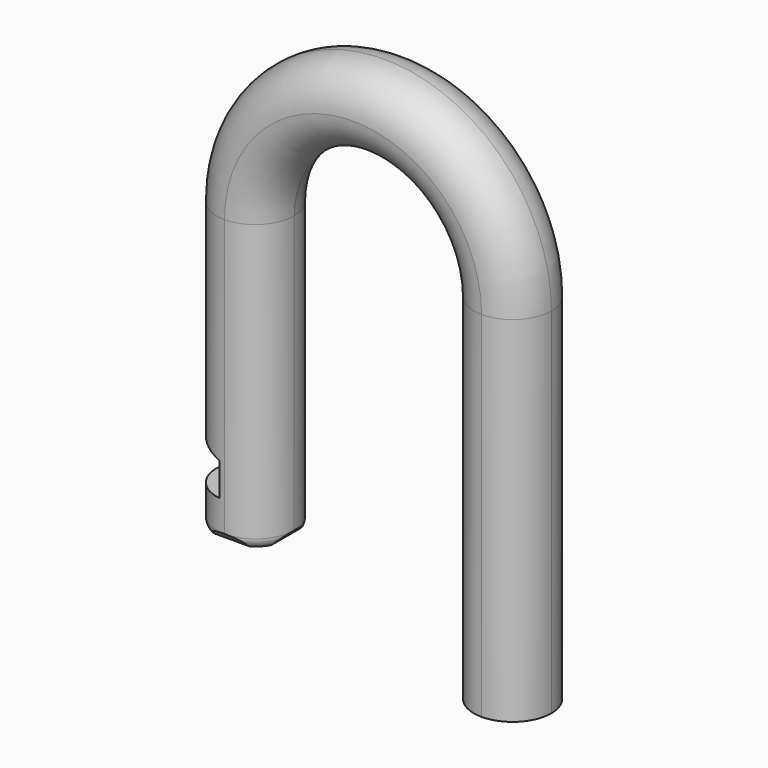
from build123d import *

# Parameters (mm, degrees)
F0_W         = 7
F0_H         = 1
F1_DEPTH     = 7
F2_SIZE      = 1
F3_T1_DEPTH  = 40.75
F3_T3_DEPTH  = 33.75
F3_T5_DEPTH  = 27.1711544693
F3_T8_ANGLE  = 180
F3_T10_ANGLE = 180
F3_T12_ANGLE = 180
F3_T14_ANGLE = 180
F4_R         = 0.99999


# Not quite as in the source:
# - a fillet or chamfer that OpenCascade refuses, or shapes differently, is made with other operations: its cross-section is extruded or revolved along the edge and cut away or added
# - a fillet or chamfer is up to 0.001 mm smaller than in the source, because OpenCascade refuses the exact size


with BuildPart() as f1:
    # F0 (on Front) → F1 (new body)
    with BuildSketch(Plane.XZ):
        with BuildLine():
            ThreePointArc((-8.115, 0), (0, 8.115), (8.115, 0))
            Line((8.115, 0), (8.115, -32))
            Line((8.115, -32), (15.115, -32))
            Line((15.115, -32), (15.115, 0))
            ThreePointArc((15.115, 0), (0, 15.115), (-15.115, 0))
            Line((-15.115, 0), (-15.115, -18.4211544693))
            Line((-15.115, -18.4211544693), (-12.115, -19.3215445876))
            Line((-12.115, -19.3215445876), (-12.115, -22.3215445876))
            Line((-12.115, -22.3215445876), (-15.115, -22.3215445876))
            Line((-15.115, -22.3215445876), (-15.115, -25))
            Line((-15.115, -25), (-8.115, -25))
            Line((-8.115, -25), (-8.115, 0))
        make_face()
        with Locations((-11.615, -25.5)):
            Rectangle(F0_W, F0_H)
    extrude(amount=-F1_DEPTH)

    # F2
    f2_edges = [f1.edges().sort_by_distance(p)[0] for p in [
        (-8.115, 3.5, -26),
        (-11.615, 0, -26),
        (-11.615, 7, -26),
        (-15.115, 3.5, -26),
    ]]
    chamfer(f2_edges, length=F2_SIZE)

    # F3: fillet of radius 3.5 on 4 edges, made by hand

    # F3_s2 → F3_t1 (cut)
    with BuildSketch(Plane.XY.offset(-40.75)):
        with BuildLine():
            ThreePointArc((11.615, 0), (9.1401262658, 1.0251262658), (8.115, 3.5))
            Line((8.115, 3.5), (8.115, 0))
            Line((8.115, 0), (11.615, 0))
        make_face()
        with BuildLine():
            ThreePointArc((11.615, 0), (14.0898737342, 1.0251262658), (15.115, 3.5))
            Line((15.115, 3.5), (15.115, 0))
            Line((15.115, 0), (11.615, 0))
        make_face()
        with BuildLine():
            ThreePointArc((11.615, 7), (14.0898737342, 5.9748737342), (15.115, 3.5))
            Line((15.115, 3.5), (15.115, 7))
            Line((15.115, 7), (11.615, 7))
        make_face()
        with BuildLine():
            ThreePointArc((11.615, 7), (9.1401262658, 5.9748737342), (8.115, 3.5))
            Line((8.115, 3.5), (8.115, 7))
            Line((8.115, 7), (11.615, 7))
        make_face()
    extrude(amount=F3_T1_DEPTH, mode=Mode.SUBTRACT)

    # F3_s4 → F3_t3 (cut)
    with BuildSketch(Plane.XY.offset(-33.75)):
        with BuildLine():
            ThreePointArc((-11.615, 7), (-9.1401262658, 5.9748737342), (-8.115, 3.5))
            Line((-8.115, 3.5), (-8.115, 7))
            Line((-8.115, 7), (-11.615, 7))
        make_face()
        with BuildLine():
            ThreePointArc((-11.615, 0), (-9.1401262658, 1.0251262658), (-8.115, 3.5))
            Line((-8.115, 3.5), (-8.115, 0))
            Line((-8.115, 0), (-11.615, 0))
        make_face()
    extrude(amount=F3_T3_DEPTH, mode=Mode.SUBTRACT)

    # F3_s6 → F3_t5 (cut)
    with BuildSketch(Plane.XY.offset(-27.1711544693)):
        with BuildLine():
            ThreePointArc((-11.615, 7), (-14.0898737342, 5.9748737342), (-15.115, 3.5))
            Line((-15.115, 3.5), (-15.115, 7))
            Line((-15.115, 7), (-11.615, 7))
        make_face()
        with BuildLine():
            ThreePointArc((-11.615, 0), (-14.0898737342, 1.0251262658), (-15.115, 3.5))
            Line((-15.115, 3.5), (-15.115, 0))
            Line((-15.115, 0), (-11.615, 0))
        make_face()
    extrude(amount=F3_T5_DEPTH, mode=Mode.SUBTRACT)

    # F3_s7 → F3_t8 (revolve, cut)
    with BuildSketch(Plane.XY):
        with BuildLine():
            ThreePointArc((-11.615, 7), (-9.1401262658, 5.9748737342), (-8.115, 3.5))
            Line((-8.115, 3.5), (-8.115, 7))
            Line((-8.115, 7), (-11.615, 7))
        make_face()
    revolve(axis=Axis((0, 7, 0), (0, 1, 0)), revolution_arc=F3_T8_ANGLE, mode=Mode.SUBTRACT)

    # F3_s9 → F3_t10 (revolve, cut)
    with BuildSketch(Plane.XY):
        with BuildLine():
            ThreePointArc((11.615, 7), (14.0898737342, 5.9748737342), (15.115, 3.5))
            Line((15.115, 3.5), (15.115, 7))
            Line((15.115, 7), (11.615, 7))
        make_face()
    revolve(axis=Axis((0, 7, 0), (0, -1, 0)), revolution_arc=F3_T10_ANGLE, mode=Mode.SUBTRACT)

    # F3_s11 → F3_t12 (revolve, cut)
    with BuildSketch(Plane.XY):
        with BuildLine():
            ThreePointArc((11.615, 0), (14.0898737342, 1.0251262658), (15.115, 3.5))
            Line((15.115, 3.5), (15.115, 0))
            Line((15.115, 0), (11.615, 0))
        make_face()
    revolve(axis=Axis((0, 0, 0), (0, -1, 0)), revolution_arc=F3_T12_ANGLE, mode=Mode.SUBTRACT)

    # F3_s13 → F3_t14 (revolve, cut)
    with BuildSketch(Plane.XY):
        with BuildLine():
            ThreePointArc((-11.615, 0), (-9.1401262658, 1.0251262658), (-8.115, 3.5))
            Line((-8.115, 3.5), (-8.115, 0))
            Line((-8.115, 0), (-11.615, 0))
        make_face()
    revolve(axis=Axis((0, 0, 0), (0, 1, 0)), revolution_arc=F3_T14_ANGLE, mode=Mode.SUBTRACT)

    # F4 (radius 1 in the source; OpenCascade refuses exactly that, so slightly less here)
    f4_edges = [f1.edges().sort_by_distance(p)[0] for p in [
        (-11.615, 6, -26),
        (-14.115, 3.5, -26),
        (-11.615, 1, -26),
        (-9.115, 3.5, -26),
        (-9.140126, 5.974874, -26),
        (-14.089874, 5.974874, -26),
        (-14.089874, 1.025126, -26),
        (-9.140126, 1.025126, -26),
    ]]
    fillet(f4_edges, radius=F4_R)


solid = f1.part
